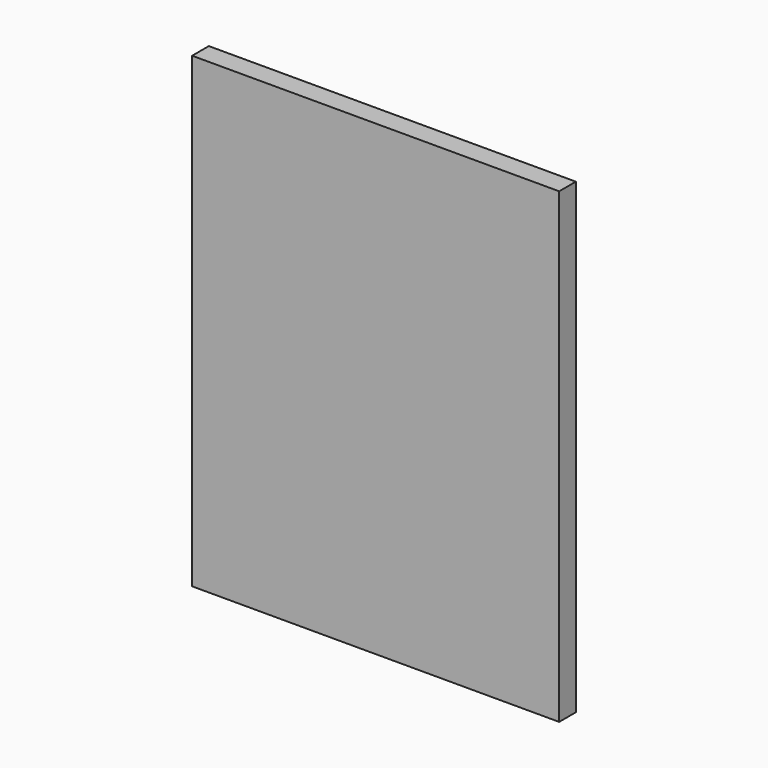
from build123d import *

# Parameters (mm, degrees)
F0_W     = 279.4
F0_H     = 355.6
F1_DEPTH = 15.875


# Not quite as in the source:
# - a length typed as a fraction of an inch, garbled in the dataset ("3 / 203.2 mm" for 3/8 in), is restored


with BuildPart() as f1:
    # F0 (on Front) → F1 (new body)
    with BuildSketch(Plane.XZ):
        with Locations((139.7, 177.8)):
            Rectangle(F0_W, F0_H)
    extrude(amount=F1_DEPTH)


solid = f1.part
